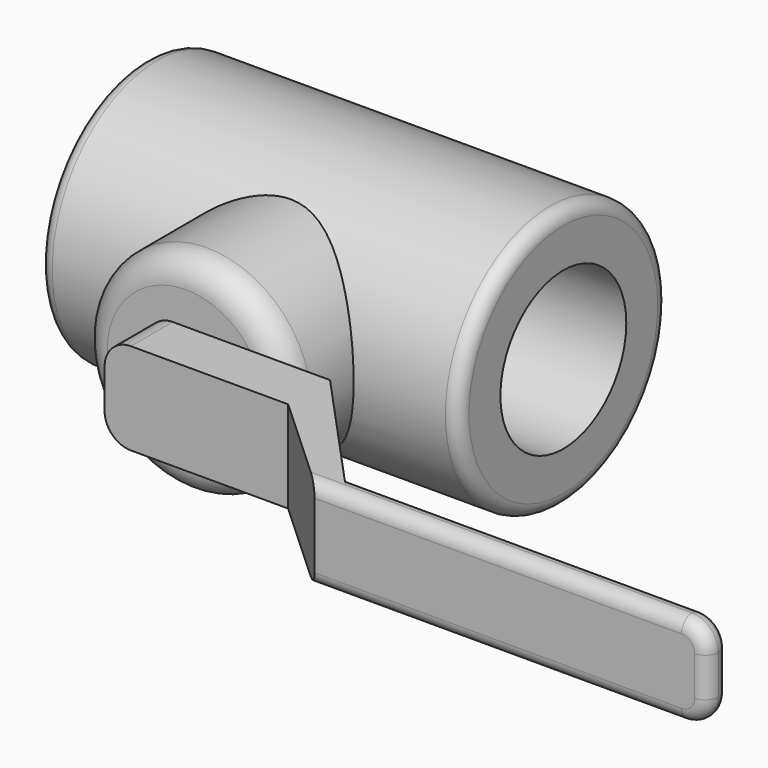
from build123d import *

# Parameters (mm, degrees)
F0_R     = 50
F0_R_2   = 30
F1_DEPTH = 160
F3_START = 30
F2_R     = 40
F3_DEPTH = 50
F4_R     = 10
F6_DEPTH = 17.5
F7_R     = 10
F8_R     = 4.99999
F9_R     = 5


# Not quite as in the source:
# - a fillet or chamfer is up to 0.001 mm smaller than in the source, because OpenCascade refuses the exact size


with BuildPart() as f1:
    # F0 (on Right) → F1 (new body)
    with BuildSketch(Plane.YZ):
        Circle(F0_R)
        Circle(F0_R_2, mode=Mode.SUBTRACT)
    extrude(amount=F1_DEPTH)

    # F2 (on Front) → F3 (join)
    with BuildSketch(Plane.XZ.offset(F3_START)):
        with Locations((80, 0)):
            Circle(F2_R)
    extrude(amount=F3_DEPTH)

    # F4
    f4_edges = [f1.edges().sort_by_distance(p)[0] for p in [
        (40, -80, 0),
    ]]
    fillet(f4_edges, radius=F4_R)

    # F5 (on Top) → F6 (join, symmetric)
    with BuildSketch(Plane.XY):
        Polygon((135, -80), (110, -80), (65, -80), (65, -100), (135, -100), (173.0335205793, -134.9323159456), (323.0335205793, -134.9323159456), (323.0335205793, -124.9323159456), (176.2279570103, -124.9323159456), align=None)
    extrude(amount=F6_DEPTH, both=True)

    # F7
    f7_edges = [f1.edges().sort_by_distance(p)[0] for p in [
        (65, -90, -17.5),
        (65, -90, 17.5),
        (323.033521, -129.932316, -17.5),
        (323.033521, -129.932316, 17.5),
    ]]
    fillet(f7_edges, radius=F7_R)

    # F8 (radius 5 in the source; OpenCascade refuses exactly that, so slightly less here)
    f8_edges = [f1.edges().sort_by_distance(p)[0] for p in [
        (243.033521, -134.932316, -17.5),
        (244.630739, -124.932316, -17.5),
    ]]
    fillet(f8_edges, radius=F8_R)

    # F9
    f9_edges = [f1.edges().sort_by_distance(p)[0] for p in [
        (160, -50, 0),
        (0, -50, 0),
    ]]
    fillet(f9_edges, radius=F9_R)


solid = f1.part
